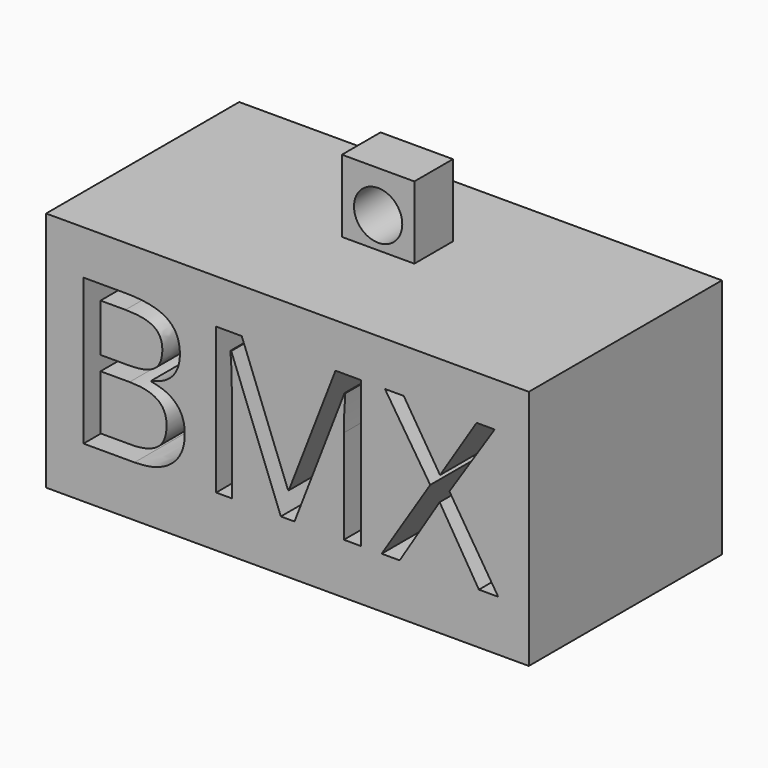
from build123d import *

# Parameters (mm, degrees)
F0_W         = 25.4
F0_H         = 12.7
F1_DEPTH     = 12.7
F2_TEXT_SIZE = 10.7695575412
F3_DEPTH     = 35.8394
F4_W         = 3.81
F4_H         = 2.54
F5_DEPTH     = 3.81
F6_R         = 1.27
F7_DEPTH     = 25.4


# Not quite as in the source:
# - Text() gives the source's letters only with a copy of the font that has no kerning and outlines rounded to 1/6400 em; it was checked with that copy


with BuildPart() as f1:
    # F0 (on Front) → F1 (new body)
    with BuildSketch(Plane.XZ):
        Rectangle(F0_W, F0_H)
    extrude(amount=F1_DEPTH)

    # F2 (on face) → F3 (cut)
    with BuildSketch(Plane.XZ.offset(12.7)):
        with Locations((-11.7867759058, -3.6679495869)):
            Text('BMX', F2_TEXT_SIZE, font='Open Sans', text_align=(TextAlign.LEFT, TextAlign.BOTTOM))
    extrude(amount=-F3_DEPTH, mode=Mode.SUBTRACT)

    # F4 (on face) → F5 (join)
    with BuildSketch(Plane.XY.offset(6.35)):
        with Locations((0, -5.4660576534)):
            Rectangle(F4_W, F4_H)
    extrude(amount=F5_DEPTH)

    # F6 (on face) → F7 (cut)
    with BuildSketch(Plane.XZ.offset(6.7360576534)):
        with Locations((0, 7.9679842228)):
            Circle(F6_R)
    extrude(amount=-F7_DEPTH, mode=Mode.SUBTRACT)


solid = f1.part
